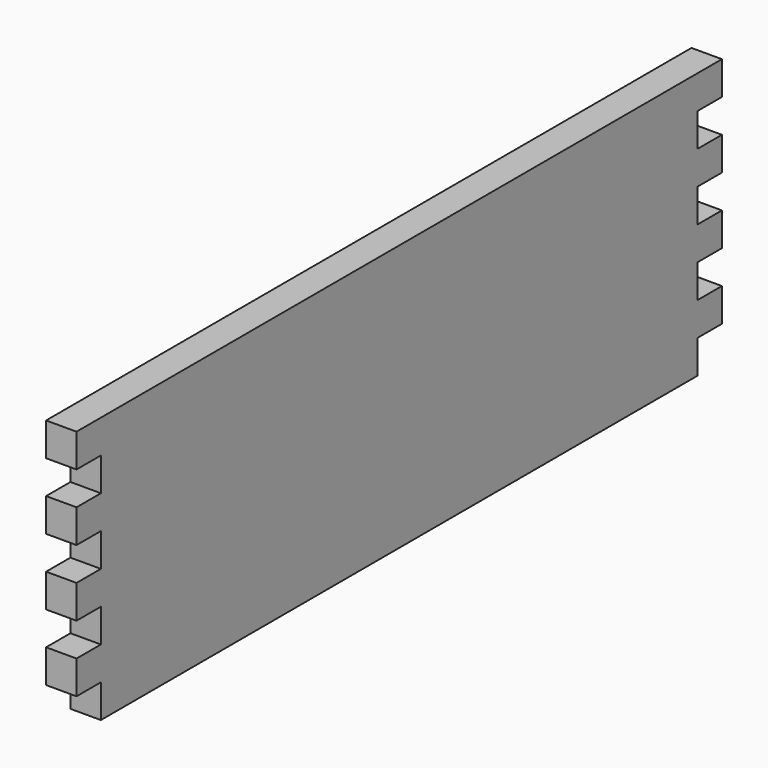
from build123d import *

# Parameters (mm, degrees)
F0_W     = 19.05
F0_H     = 166.624
F1_DEPTH = 252.4125
F3_W     = 19.05
F3_H     = 20.828
F4_DEPTH = 19.051
F7_R     = 101.6
F8_DEPTH = 10.4902


# Not quite as in the source:
# - a length typed as a fraction of an inch, garbled in the dataset ("3 / 203.2 mm" for 3/8 in), is restored


with BuildPart() as f1:
    # F0 (on Front) → F1 (new body)
    with BuildSketch(Plane.XZ):
        with Locations((-9.525, 83.312)):
            Rectangle(F0_W, F0_H)
    extrude(amount=-F1_DEPTH)

    # F3 (on Right) → F4 (cut, through all)
    with BuildSketch(Plane.YZ):
        with Locations((9.525, 135.382)):
            Rectangle(F3_W, F3_H)
        with Locations((9.525, 93.726)):
            Rectangle(F3_W, F3_H)
        with Locations((9.525, 52.07)):
            Rectangle(F3_W, F3_H)
        with Locations((9.525, 10.414)):
            Rectangle(F3_W, F3_H)
    extrude(amount=-F4_DEPTH, mode=Mode.SUBTRACT)

    # F5: F1 across face


with BuildPart() as f1_1:
    add(f1.part)
    add(f1.part.mirror(Plane(origin=(-9.525, 252.4125, 83.312), x_dir=(1, 0, 0), z_dir=(0, 1, 0))))

    # F7 (on offset) → F8 (cut, symmetric)
    with BuildSketch(Plane.XY.offset(76.2)):
        with Locations((-111.125, 252.4125)):
            Circle(F7_R)
    extrude(amount=F8_DEPTH, both=True, mode=Mode.SUBTRACT)


solid = f1_1.part
